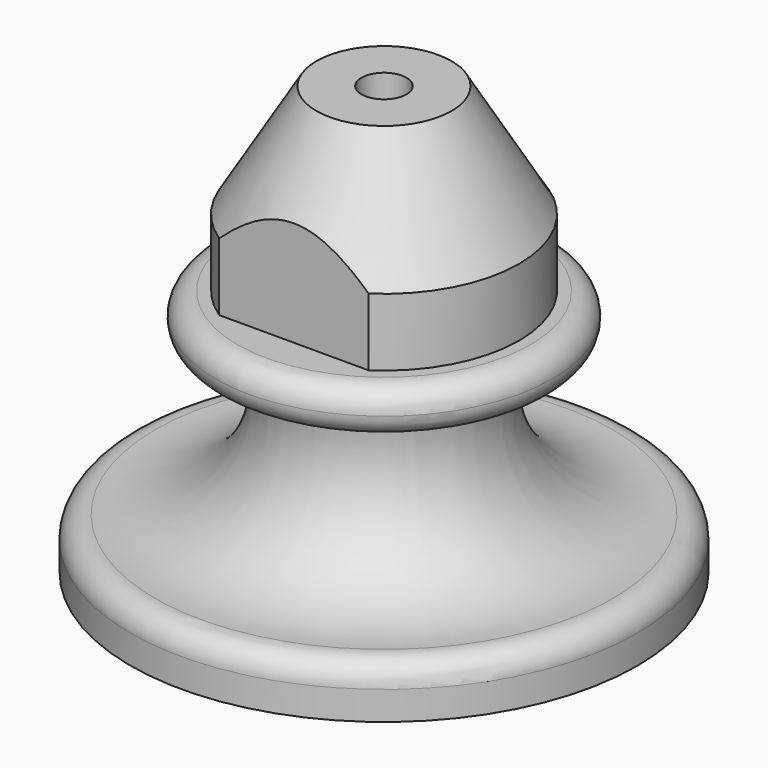
from build123d import *

# Parameters (mm, degrees)
F2_R     = 2
F3_R     = 1.99999
F5_DEPTH = 16


# Not quite as in the source:
# - a fillet or chamfer is up to 0.001 mm smaller than in the source, because OpenCascade refuses the exact size


with BuildPart() as f1:
    # F0 (on Front) → F1 (revolve)
    with BuildSketch(Plane.XZ):
        with BuildLine():
            Line((-2, 25), (-2, 38))
            Line((-2, 38), (-6, 38))
            Line((-6, 38), (-12, 28))
            Line((-12, 28), (-12, 22))
            Line((-12, 22), (-15, 22))
            Line((-15, 22), (-15, 18))
            Line((-15, 18), (-11.5086935796, 18))
            ThreePointArc((-11.5086935796, 18), (-10.2343072055, 17.5414082423), (-9.5443439187, 16.3759393693))
            ThreePointArc((-9.5443439187, 16.3759393693), (-11.9690635692, 7.766906219), (-20.3110153706, 4.540986612))
            ThreePointArc((-20.3110153706, 4.540986612), (-21.8457397113, 4.0294571869), (-22.5, 2.5499354299))
            Line((-22.5, 2.5499354299), (-22.5, 0))
            Line((-22.5, 0), (-19.5, 0))
            ThreePointArc((-19.5, 0), (-19.029745792, 1.2883624536), (-17.8401221881, 1.970867042))
            ThreePointArc((-17.8401221881, 1.970867042), (-9.6957329077, 6.4947102095), (-7, 15.4126280071))
            Line((-7, 15.4126280071), (-7, 23))
            ThreePointArc((-7, 23), (-6.4142135624, 24.4142135624), (-5, 25))
            Line((-5, 25), (-2, 25))
        make_face()
    revolve(axis=Axis((0, 0, 32.4923060834), (0, 0, -1)))

    # F2
    f2_edges = [f1.edges().sort_by_distance(p)[0] for p in [
        (15, 0, 22),
    ]]
    fillet(f2_edges, radius=F2_R)

    # F3 (radius 2 in the source; OpenCascade refuses exactly that, so slightly less here)
    f3_edges = [f1.edges().sort_by_distance(p)[0] for p in [
        (15, 0, 18),
    ]]
    fillet(f3_edges, radius=F3_R)

    # F4 (on face) → F5 (cut)
    with BuildSketch(Plane.XY.offset(38)):
        with BuildLine():
            Line((-6.6332495807, 10), (6.6332495807, 10))
            ThreePointArc((6.6332495807, 10), (0, 12), (-6.6332495807, 10))
        make_face()
        with BuildLine():
            ThreePointArc((-6.6332495807, -10), (0, -12), (6.6332495807, -10))
            Line((6.6332495807, -10), (-6.6332495807, -10))
        make_face()
    extrude(amount=-F5_DEPTH, mode=Mode.SUBTRACT)


solid = f1.part
